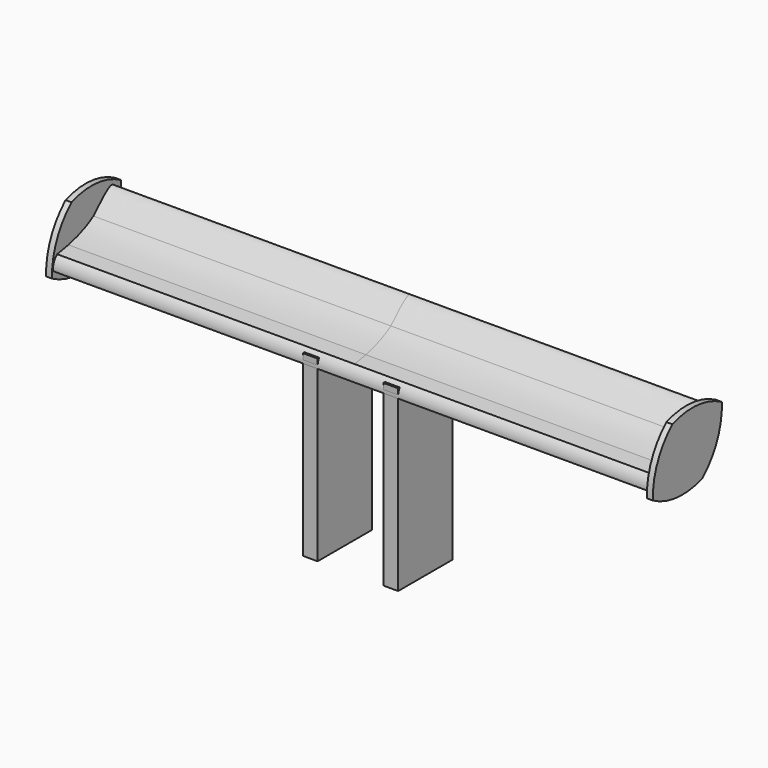
from build123d import *

# Parameters (mm, degrees)
F1_DEPTH    = 254
F3_DEPTH    = 5.08
F4_W        = 12.6729309559
F4_H        = 57.9334199429
F5_DEPTH    = 152.4
F6_T1_DEPTH = 319.230203427


# Not quite as in the source:
# - a fillet or chamfer that OpenCascade refuses, or shapes differently, is made with other operations: its cross-section is extruded or revolved along the edge and cut away or added


with BuildPart() as f1:
    # F0 (on Right) → F1 (new body)
    with BuildSketch(Plane.YZ):
        with BuildLine():
            ThreePointArc((-24.5272097082, 3.183184572), (-28.1195399904, -1.6994877312), (-28.9857762817, -7.6990677469))
            ThreePointArc((-28.9857762817, -7.6990677469), (7.8240128757, -12.8494213203), (33.8808850254, 13.655788234))
            add(Edge.make_bspline(
                [(14.1425715482, 16.1532932262), (25.4105223066, 27.4543127656), (43.1557495947, 45.6951015007), (33.8808850254, 13.655788234)],
                knots=[0, 0, 0, 0, 19.8956917475, 19.8956917475, 19.8956917475, 19.8956917475], degree=3))
            add(Edge.make_bspline(
                [(-12.5656056095, 5.3816662895), (-2.2918152978, 7.5478072589), (6.5829970209, 11.1284464372), (14.1425715482, 16.1532932262)],
                knots=[0, 0, 0, 0, 28.7985186069, 28.7985186069, 28.7985186069, 28.7985186069], degree=3))
            add(Edge.make_bspline(
                [(-24.5272097082, 3.183184572), (-21.1546527218, 3.8161453558), (-17.1728906965, 4.5318009653), (-12.5656056095, 5.3816662895)],
                knots=[17.6782467535, 17.6782467535, 17.6782467535, 17.6782467535, 20.9935134705, 20.9935134705, 20.9935134705, 20.9935134705], degree=3))
        make_face()
    extrude(amount=F1_DEPTH)

    # F7: F1, F3, F5 across face


with BuildPart() as f3:
    # F2 (on face) → F3 (new body)
    with BuildSketch(Plane.YZ.offset(254)):
        Polygon((33.7327011203, 63.0955714471), (-53.4129644445, 10.863464719), (-20.0576754131, -44.7875331985), (67.0879901518, 7.4445735296), align=None)
    extrude(amount=F3_DEPTH)

    # F6: fillet of radius 62.8300406854 on 4 edges, made by hand

    # F6_s2 → F6_t1 (cut)
    with BuildSketch(Plane.YZ.offset(96.9248982865)):
        with BuildLine():
            ThreePointArc((33.8337193999, -12.4868895882), (-13.7338907968, -19.5424696286), (-52.3583190234, 9.1038616144))
            Line((-52.3583190234, 9.1038616144), (-20.0576754131, -44.7875331985))
            Line((-20.0576754131, -44.7875331985), (33.8337193999, -12.4868895882))
        make_face()
        with BuildLine():
            ThreePointArc((0.4784303684, 43.1641083293), (-28.1679008746, 4.5396801026), (-21.1123208342, -43.027930094))
            Line((-21.1123208342, -43.027930094), (-53.4129644445, 10.863464719))
            Line((-53.4129644445, 10.863464719), (0.4784303684, 43.1641083293))
        make_face()
        with BuildLine():
            ThreePointArc((66.0333447307, 9.2041766341), (27.408916504, 37.8505078772), (-20.1586936926, 30.7949278367))
            Line((-20.1586936926, 30.7949278367), (33.7327011203, 63.0955714471))
            Line((33.7327011203, 63.0955714471), (66.0333447307, 9.2041766341))
        make_face()
        with BuildLine():
            ThreePointArc((13.1965953388, -24.8560700808), (41.8429265819, 13.7683581459), (34.7873465414, 61.3359683426))
            Line((34.7873465414, 61.3359683426), (67.0879901518, 7.4445735296))
            Line((67.0879901518, 7.4445735296), (13.1965953388, -24.8560700808))
        make_face()
    extrude(amount=F6_T1_DEPTH, mode=Mode.SUBTRACT)


with BuildPart() as f5:
    # F4 (on Top) → F5 (new body)
    with BuildSketch(Plane.XY):
        with Locations((34.3979746103, 0)):
            Rectangle(F4_W, F4_H)
    extrude(amount=-F5_DEPTH)


with BuildPart() as f1_1:
    add(f1.part)
    add(f1.part.mirror(Plane(origin=(0, 6.6636224676, 3.2061249458), x_dir=(0, 1, 0), z_dir=(-1, 0, 0))))
    add(f3.part.mirror(Plane(origin=(0, 6.6636224676, 3.2061249458), x_dir=(0, 1, 0), z_dir=(-1, 0, 0))))
    add(f5.part.mirror(Plane(origin=(0, 6.6636224676, 3.2061249458), x_dir=(0, 1, 0), z_dir=(-1, 0, 0))))


solid = Compound([f3.part, f5.part, f1_1.part])
